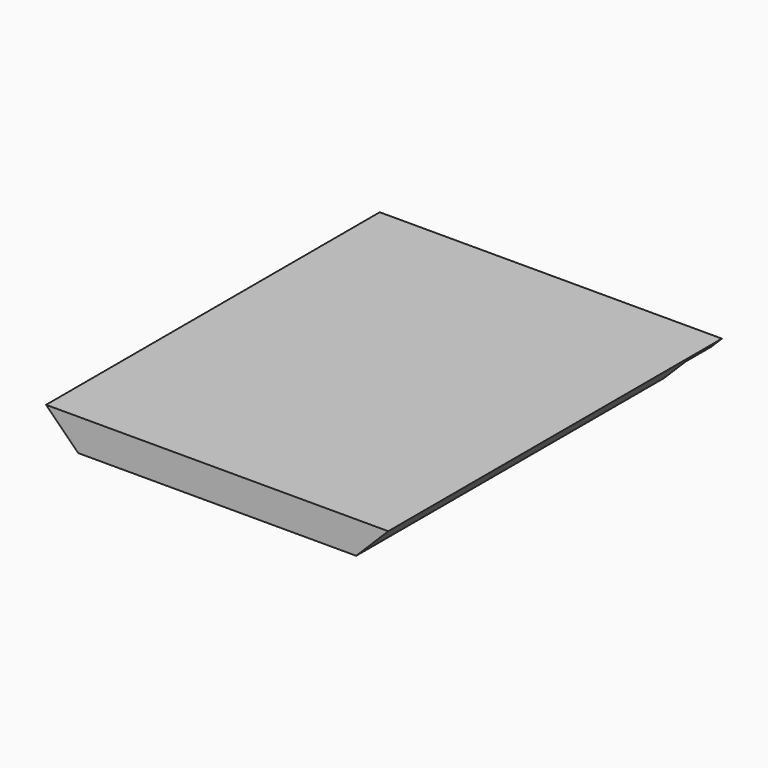
from build123d import *

# Parameters (mm, degrees)
F0_W     = 203.2
F0_H     = 247.65
F1_DEPTH = 19.05
F2_W     = 19.05
F2_H     = 12.7
F3_DEPTH = 203.201
F4_SIZE  = 19.04999
F5_SIZE  = 19.04999


# Not quite as in the source:
# - a fillet or chamfer is up to 0.001 mm smaller than in the source, because OpenCascade refuses the exact size


with BuildPart() as f1:
    # F0 (on Top) → F1 (new body)
    with BuildSketch(Plane.XY):
        Rectangle(F0_W, F0_H)
    extrude(amount=F1_DEPTH)

    # F2 (on face) → F3 (cut, through all)
    with BuildSketch(Plane(origin=(-101.6, 0, 0), x_dir=(0, -1, 0), z_dir=(-1, 0, 0))):
        with Locations((-114.3, 6.35)):
            Rectangle(F2_W, F2_H)
    extrude(amount=-F3_DEPTH, mode=Mode.SUBTRACT)

    # F4 (size 19.05 in the source; OpenCascade refuses exactly that, so slightly less here)
    f4_edges = [f1.edges().sort_by_distance(p)[0] for p in [
        (-101.6, -9.525, 0),
    ]]
    chamfer(f4_edges, length=F4_SIZE)

    # F5 (size 19.05 in the source; OpenCascade refuses exactly that, so slightly less here)
    f5_edges = [f1.edges().sort_by_distance(p)[0] for p in [
        (101.6, -9.525, 0),
    ]]
    chamfer(f5_edges, length=F5_SIZE)


solid = f1.part
